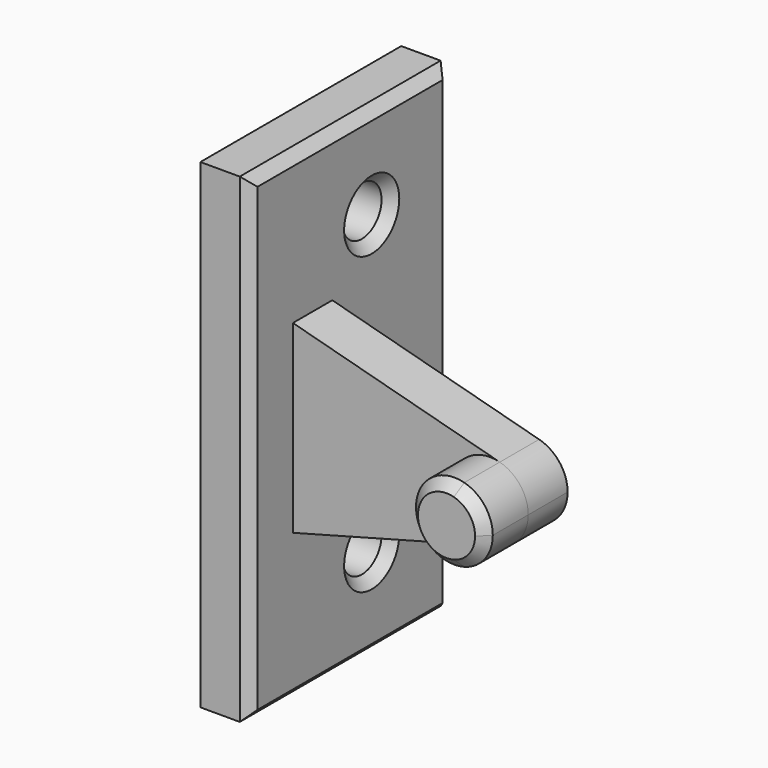
from build123d import *

# Parameters (mm, degrees)
F1_DEPTH  = 5.5
F2_DEPTH  = 5
F3_DEPTH  = 20
F4_R      = 2.5
F5_DEPTH  = 10
F6_SIZE   = 1
F6_2_SIZE = 1


with BuildPart() as f1:
    # F0 (on Front) → F1 (new body)
    with BuildSketch(Plane.XZ):
        with BuildLine():
            ThreePointArc((1.0068716538, -3.767785752), (3.0932830011, -2.3752053122), (3.9, 0))
            ThreePointArc((3.9, 0), (3.0932830011, 2.3752053122), (1.0068716538, 3.767785752))
            ThreePointArc((1.0068716538, 3.767785752), (-3.9, 0), (1.0068716538, -3.767785752))
        make_face()
    extrude(amount=F1_DEPTH)

    # F0 (on Front) → F2 (join)
    with BuildSketch(Plane.XZ):
        with BuildLine():
            ThreePointArc((1.0068716538, -3.767785752), (-3.9, 0), (1.0068716538, 3.767785752))
            Line((1.0068716538, 3.767785752), (-20, 9.3814870065))
            Line((-20, 9.3814870065), (-20, 0))
            Line((-20, 0), (-20, -9.3814870065))
            Line((-20, -9.3814870065), (1.0068716538, -3.767785752))
        make_face()
        with BuildLine():
            ThreePointArc((1.0068716538, -3.767785752), (3.0932830011, -2.3752053122), (3.9, 0))
            ThreePointArc((3.9, 0), (3.0932830011, 2.3752053122), (1.0068716538, 3.767785752))
            ThreePointArc((1.0068716538, 3.767785752), (-3.9, 0), (1.0068716538, -3.767785752))
        make_face()
    extrude(amount=-F2_DEPTH)

    # F6
    f6_edges = [f1.edges().sort_by_distance(p)[0] for p in [
        (-1.006872, -5.5, 3.767786),
    ]]
    chamfer(f6_edges, length=F6_SIZE)


with BuildPart() as f1b:
    # F0 (on Front) → F1, piece 2 (new body)
    with BuildSketch(Plane.XZ):
        Polygon((-20, 0), (-20, 9.3814870065), (-20, 24.3814870065), (-25, 24.3814870065), (-25, 0.7844285667), (-25, -9.3814870065), (-25, -24.3814870065), (-20, -24.3814870065), (-20, -9.3814870065), align=None)
    extrude(amount=F1_DEPTH)

    # F0 (on Front) → F3 (join)
    with BuildSketch(Plane.XZ):
        Polygon((-20, 0), (-20, 9.3814870065), (-20, 24.3814870065), (-25, 24.3814870065), (-25, 0.7844285667), (-25, -9.3814870065), (-25, -24.3814870065), (-20, -24.3814870065), (-20, -9.3814870065), align=None)
    extrude(amount=-F3_DEPTH)

    # F4 (on face) → F5 (cut)
    with BuildSketch(Plane.YZ.offset(-20)):
        with Locations((10, 15)):
            Circle(F4_R)
        with Locations((10, -15)):
            Circle(F4_R)
    extrude(amount=-F5_DEPTH, mode=Mode.SUBTRACT)

    # F6#2
    f6_2_edges = [f1b.edges().sort_by_distance(p)[0] for p in [
        (-20, 7.5, 15),
        (-20, 7.5, -15),
        (-20, 20, 0),
        (-20, 7.25, 24.381487),
        (-20, -5.5, 0),
        (-20, 7.25, -24.381487),
    ]]
    chamfer(f6_2_edges, length=F6_2_SIZE)


solid = Compound([f1.part, f1b.part])
